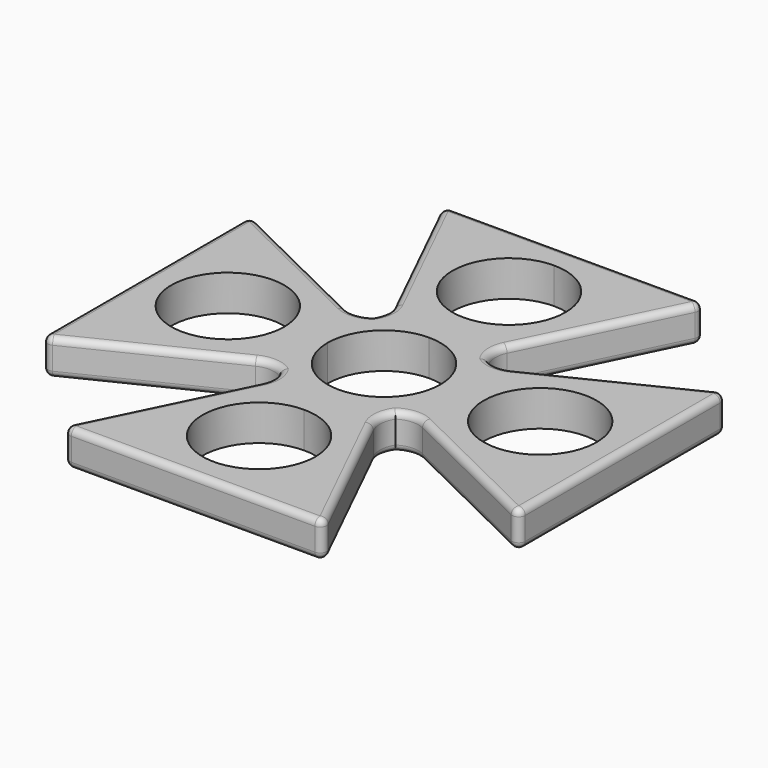
from build123d import *

# Parameters (mm, degrees)
F0_R          = 11.0109
F1_DEPTH      = 6.985
F2_R          = 1.27
F3_T1_DEPTH   = 6.985
F4_T1_DEPTH   = 47.5314771429
F4_T3_DEPTH   = 31.6719082331
F4_T5_DEPTH   = 31.6719082331
F4_T7_DEPTH   = 31.6719082331
F4_T9_DEPTH   = 47.5314771429
F4_T11_DEPTH  = 31.6719082331
F4_T13_DEPTH  = 31.6719082331
F4_T15_DEPTH  = 31.6719082331
F4_T17_DEPTH  = 31.6719082331
F4_T19_DEPTH  = 31.6719082331
F4_T22_ANGLE  = 116.1026378833
F4_T26_ANGLE  = 95.1309457851
F4_T31_ANGLE  = 95.1309457851
F4_S32_R      = 5.0800000002
F4_T33_DEPTH  = 7
F4_T35_ANGLE  = 116.1026378833
F4_T39_ANGLE  = 95.1309457851
F4_T44_ANGLE  = 95.1309457851
F4_S45_R      = 5.0800000002
F4_T46_DEPTH  = 8
F4_T48_ANGLE  = 116.1026378833
F4_T52_ANGLE  = 95.1309457851
F4_T57_ANGLE  = 95.1309457851
F4_S58_R      = 5.0800000002
F4_T59_DEPTH  = 8
F4_T61_ANGLE  = 116.1026378833
F4_T65_ANGLE  = 95.1309457851
F4_S66_R      = 5.0800000002
F4_T67_DEPTH  = 7
F4_T71_ANGLE  = 95.1309457851
F4_T76_ANGLE  = 95.1309457851
F4_S77_R      = 5.0800000002
F4_T78_DEPTH  = 8
F4_T82_ANGLE  = 95.1309457851
F4_T85_ANGLE  = 116.1026378833
F4_T87_ANGLE  = 116.1026378833
F4_T91_ANGLE  = 95.1309457851
F4_S92_R      = 5.0800000002
F4_T93_DEPTH  = 8
F4_T97_ANGLE  = 95.1309457851
F4_T100_ANGLE = 116.1026378833
F4_T102_ANGLE = 116.1026378833
F4_T106_ANGLE = 95.1309457851
F4_S107_R     = 5.0800000002
F4_T108_DEPTH = 8
F4_T112_ANGLE = 95.1309457851
F4_T117_ANGLE = 95.1309457851
F4_T122_ANGLE = 95.1309457851
F4_S123_R     = 5.0800000002
F4_T124_DEPTH = 8
F4_T129_ANGLE = 95.1309457851
F4_S131_R     = 5.0800000002
F4_T132_DEPTH = 7
F4_T135_ANGLE = 95.1309457851
F4_S137_R     = 5.0800000002
F4_T138_DEPTH = 7
F4_T144_ANGLE = 95.1309457851
F4_S145_R     = 5.0800000002
F4_T146_DEPTH = 8
F4_T150_ANGLE = 95.1309457851
F4_S152_R     = 5.0800000002
F4_T153_DEPTH = 8
F4_T159_ANGLE = 95.1309457851
F4_S161_R     = 5.0800000002
F4_T162_DEPTH = 8
F4_T165_ANGLE = 95.1309457851
F4_S167_R     = 5.0800000002
F4_T168_DEPTH = 8
F4_T174_ANGLE = 95.1309457851
F4_S176_R     = 5.0800000002
F4_T177_DEPTH = 8
F4_T180_ANGLE = 95.1309457851
F4_S182_R     = 5.0800000002
F4_T183_DEPTH = 8
F5_T1_DEPTH   = 31.6719082331
F5_T3_DEPTH   = 31.6719082331
F5_T5_DEPTH   = 31.6719082331
F5_T7_DEPTH   = 31.6719082331
F5_T9_DEPTH   = 47.5314771429
F5_T11_DEPTH  = 31.6719082331
F5_T13_DEPTH  = 31.6719082331
F5_T15_DEPTH  = 47.5314771429
F5_T17_DEPTH  = 31.6719082331
F5_T19_DEPTH  = 31.6719082331
F5_T22_ANGLE  = 116.1026378833
F5_T26_ANGLE  = 95.1309457851
F5_T31_ANGLE  = 95.1309457851
F5_S32_R      = 5.0800000002
F5_T33_DEPTH  = 8
F5_T35_ANGLE  = 116.1026378833
F5_T39_ANGLE  = 95.1309457851
F5_T44_ANGLE  = 95.1309457851
F5_S45_R      = 5.0800000002
F5_T46_DEPTH  = 8
F5_T48_ANGLE  = 116.1026378833
F5_T52_ANGLE  = 95.1309457851
F5_S53_R      = 5.0800000002
F5_T54_DEPTH  = 8
F5_T58_ANGLE  = 95.1309457851
F5_T63_ANGLE  = 95.1309457851
F5_T68_ANGLE  = 95.1309457851
F5_S69_R      = 5.0800000002
F5_T70_DEPTH  = 8
F5_T72_ANGLE  = 116.1026378833
F5_T74_ANGLE  = 116.1026378833
F5_T78_ANGLE  = 95.1309457851
F5_S79_R      = 5.0800000002
F5_T80_DEPTH  = 8
F5_T84_ANGLE  = 95.1309457851
F5_T89_ANGLE  = 95.1309457851
F5_T94_ANGLE  = 95.1309457851
F5_S95_R      = 5.0800000002
F5_T96_DEPTH  = 8
F5_T98_ANGLE  = 116.1026378833
F5_T102_ANGLE = 95.1309457851
F5_S103_R     = 5.0800000002
F5_T104_DEPTH = 8
F5_T108_ANGLE = 95.1309457851
F5_T111_ANGLE = 116.1026378833
F5_T115_ANGLE = 95.1309457851
F5_S116_R     = 5.0800000002
F5_T117_DEPTH = 8
F5_T121_ANGLE = 95.1309457851
F5_T124_ANGLE = 116.1026378833
F5_T129_ANGLE = 95.1309457851
F5_S131_R     = 5.0800000002
F5_T132_DEPTH = 8
F5_T135_ANGLE = 95.1309457851
F5_S136_R     = 5.0800000002
F5_T137_DEPTH = 8
F5_T144_ANGLE = 95.1309457851
F5_S146_R     = 5.0800000002
F5_T147_DEPTH = 8
F5_T150_ANGLE = 95.1309457851
F5_S151_R     = 5.0800000002
F5_T152_DEPTH = 8
F5_T159_ANGLE = 95.1309457851
F5_S160_R     = 5.0800000002
F5_T161_DEPTH = 8
F5_T165_ANGLE = 95.1309457851
F5_S166_R     = 5.0800000002
F5_T167_DEPTH = 8
F5_T174_ANGLE = 95.1309457851
F5_S176_R     = 5.0800000002
F5_T177_DEPTH = 8
F5_T180_ANGLE = 95.1309457851
F5_S181_R     = 5.0800000002
F5_T182_DEPTH = 8


# Not quite as in the source:
# - a fillet or chamfer that OpenCascade refuses, or shapes differently, is made with other operations: its cross-section is extruded or revolved along the edge and cut away or added


with BuildPart() as f1:
    # F0 (on Top) → F1 (new body)
    with BuildSketch(Plane.XY):
        with BuildLine():
            Line((15.875, 0), (11.0109, 0))
            ThreePointArc((11.0109, 0), (7.785882057, -7.785882057), (0, -11.0109))
            Line((0, -11.0109), (0, -15.875))
            ThreePointArc((0, -15.875), (4.8823009597, -15.1055871233), (9.2913414184, -12.8719306884))
            ThreePointArc((9.2913414184, -12.8719306884), (11.2253201513, -11.2253201513), (12.8719306884, -9.2913414184))
            ThreePointArc((12.8719306884, -9.2913414184), (15.1055871233, -4.8823009597), (15.875, 0))
        make_face()
        with BuildLine():
            ThreePointArc((0, 11.0109), (7.785882057, 7.785882057), (11.0109, 0))
            Line((11.0109, 0), (15.875, 0))
            ThreePointArc((15.875, 0), (15.1055871233, 4.8823009597), (12.8719306884, 9.2913414184))
            ThreePointArc((12.8719306884, 9.2913414184), (11.2253201513, 11.2253201513), (9.2913414184, 12.8719306884))
            ThreePointArc((9.2913414184, 12.8719306884), (4.8823009597, 15.1055871233), (0, 15.875))
            Line((0, 15.875), (0, 11.0109))
        make_face()
        with BuildLine():
            ThreePointArc((-11.0109, 0), (-7.785882057, 7.785882057), (0, 11.0109))
            Line((0, 11.0109), (0, 15.875))
            ThreePointArc((0, 15.875), (-4.8823009597, 15.1055871233), (-9.2913414184, 12.8719306884))
            ThreePointArc((-9.2913414184, 12.8719306884), (-11.2253201513, 11.2253201513), (-12.8719306884, 9.2913414184))
            ThreePointArc((-12.8719306884, 9.2913414184), (-15.1055871233, 4.8823009597), (-15.875, 0))
            Line((-15.875, 0), (-11.0109, 0))
        make_face()
        with BuildLine():
            Line((0, -15.875), (0, -11.0109))
            ThreePointArc((0, -11.0109), (-4.2136890054, -10.1727451445), (-7.785882057, -7.785882057))
            Line((-7.785882057, -7.785882057), (-11.2253201513, -11.2253201513))
            ThreePointArc((-11.2253201513, -11.2253201513), (-10.2913158565, -12.0873670807), (-9.2913414184, -12.8719306884))
            ThreePointArc((-9.2913414184, -12.8719306884), (-4.8823009597, -15.1055871233), (0, -15.875))
        make_face()
        with BuildLine():
            ThreePointArc((12.8719306884, 9.2913414184), (15.1055871233, 4.8823009597), (15.875, 0))
            ThreePointArc((15.875, 0), (15.1055871233, -4.8823009597), (12.8719306884, -9.2913414184))
            Line((12.8719306884, -9.2913414184), (46.5709, -25.8022200257))
            Line((46.5709, -25.8022200257), (46.5709, 25.8022200257))
            Line((46.5709, 25.8022200257), (12.8719306884, 9.2913414184))
        make_face()
        with BuildLine():
            ThreePointArc((41.4909, 0), (30.48, -11.0109), (19.4691, 0))
            ThreePointArc((19.4691, 0), (30.48, 11.0109), (41.4909, 0))
        make_face(mode=Mode.SUBTRACT)
        with BuildLine():
            ThreePointArc((-7.785882057, -7.785882057), (-10.1727451445, -4.2136890054), (-11.0109, 0))
            Line((-11.0109, 0), (-15.875, 0))
            ThreePointArc((-15.875, 0), (-15.1055871233, -4.8823009597), (-12.8719306884, -9.2913414184))
            ThreePointArc((-12.8719306884, -9.2913414184), (-12.0873670807, -10.2913158565), (-11.2253201513, -11.2253201513))
            Line((-11.2253201513, -11.2253201513), (-7.785882057, -7.785882057))
        make_face()
        with BuildLine():
            ThreePointArc((-9.2913414184, 12.8719306884), (-4.8823009597, 15.1055871233), (0, 15.875))
            Line((0, 15.875), (0, 19.4691))
            ThreePointArc((0, 19.4691), (-11.0109, 30.48), (0, 41.4909))
            Line((0, 41.4909), (0, 46.5709))
            Line((0, 46.5709), (-25.8022200257, 46.5709))
            Line((-25.8022200257, 46.5709), (-9.2913414184, 12.8719306884))
        make_face()
        with BuildLine():
            Line((0, 19.4691), (0, 15.875))
            ThreePointArc((0, 15.875), (4.8823009597, 15.1055871233), (9.2913414184, 12.8719306884))
            Line((9.2913414184, 12.8719306884), (25.8022200257, 46.5709))
            Line((25.8022200257, 46.5709), (0, 46.5709))
            Line((0, 46.5709), (0, 41.4909))
            ThreePointArc((0, 41.4909), (7.785882057, 38.265882057), (11.0109, 30.48))
            ThreePointArc((11.0109, 30.48), (7.785882057, 22.694117943), (0, 19.4691))
        make_face()
        with BuildLine():
            ThreePointArc((9.2913414184, -12.8719306884), (4.8823009597, -15.1055871233), (0, -15.875))
            ThreePointArc((0, -15.875), (-4.8823009597, -15.1055871233), (-9.2913414184, -12.8719306884))
            Line((-9.2913414184, -12.8719306884), (-25.8022200257, -46.5709))
            Line((-25.8022200257, -46.5709), (25.8022200257, -46.5709))
            Line((25.8022200257, -46.5709), (9.2913414184, -12.8719306884))
        make_face()
        with BuildLine():
            ThreePointArc((11.0109, -30.48), (-7.785882057, -38.265882057), (0, -19.4691))
            ThreePointArc((0, -19.4691), (7.785882057, -22.694117943), (11.0109, -30.48))
        make_face(mode=Mode.SUBTRACT)
        with BuildLine():
            ThreePointArc((-12.8719306884, -9.2913414184), (-15.1055871233, -4.8823009597), (-15.875, 0))
            ThreePointArc((-15.875, 0), (-15.1055871233, 4.8823009597), (-12.8719306884, 9.2913414184))
            Line((-12.8719306884, 9.2913414184), (-46.5709, 25.8022200257))
            Line((-46.5709, 25.8022200257), (-46.5709, -25.8022200257))
            Line((-46.5709, -25.8022200257), (-12.8719306884, -9.2913414184))
        make_face()
        with Locations((-30.48, 0)):
            Circle(F0_R, mode=Mode.SUBTRACT)
    extrude(amount=F1_DEPTH)

    # F2
    f2_edges = [f1.edges().sort_by_distance(p)[0] for p in [
        (-25.80222, 46.5709, 3.4925),
        (-46.5709, 25.80222, 3.4925),
        (25.80222, 46.5709, 3.4925),
        (46.5709, 25.80222, 3.4925),
        (-46.5709, -25.80222, 3.4925),
        (-25.80222, -46.5709, 3.4925),
        (25.80222, -46.5709, 3.4925),
        (46.5709, -25.80222, 3.4925),
    ]]
    fillet(f2_edges, radius=F2_R)

    # F3: fillet of radius 5.08 on 8 edges, made by hand

    # F3_s2 → F3_t1 (join)
    with BuildSketch(Plane.XY):
        with BuildLine():
            ThreePointArc((11.7674716509, 10.655619923), (10.5028634206, 13.3558434789), (10.971185393, 16.3005193113))
            Line((10.971185393, 16.3005193113), (9.2913414184, 12.8719306884))
            ThreePointArc((9.2913414184, 12.8719306884), (10.5875592241, 11.8287452705), (11.7674716509, 10.655619923))
        make_face()
        with BuildLine():
            ThreePointArc((16.3005193113, 10.971185393), (13.3558434789, 10.5028634206), (10.655619923, 11.7674716509))
            ThreePointArc((10.655619923, 11.7674716509), (11.8287452705, 10.5875592241), (12.8719306884, 9.2913414184))
            Line((12.8719306884, 9.2913414184), (16.3005193113, 10.971185393))
        make_face()
        with BuildLine():
            ThreePointArc((16.3005193113, -10.971185393), (13.3558434789, -10.5028634206), (10.655619923, -11.7674716509))
            ThreePointArc((10.655619923, -11.7674716509), (11.8287452705, -10.5875592241), (12.8719306884, -9.2913414184))
            Line((12.8719306884, -9.2913414184), (16.3005193113, -10.971185393))
        make_face()
        with BuildLine():
            ThreePointArc((11.7674716509, -10.655619923), (10.5028634206, -13.3558434789), (10.971185393, -16.3005193113))
            Line((10.971185393, -16.3005193113), (9.2913414184, -12.8719306884))
            ThreePointArc((9.2913414184, -12.8719306884), (10.5875592241, -11.8287452705), (11.7674716509, -10.655619923))
        make_face()
        with BuildLine():
            ThreePointArc((-10.971185393, -16.3005193113), (-10.5028634206, -13.3558434789), (-11.7674716509, -10.655619923))
            ThreePointArc((-11.7674716509, -10.655619923), (-10.5875592241, -11.8287452705), (-9.2913414184, -12.8719306884))
            Line((-9.2913414184, -12.8719306884), (-10.971185393, -16.3005193113))
        make_face()
        with BuildLine():
            ThreePointArc((-10.655619923, -11.7674716509), (-13.3558434789, -10.5028634206), (-16.3005193113, -10.971185393))
            Line((-16.3005193113, -10.971185393), (-12.8719306884, -9.2913414184))
            ThreePointArc((-12.8719306884, -9.2913414184), (-11.8287452705, -10.5875592241), (-10.655619923, -11.7674716509))
        make_face()
        with BuildLine():
            ThreePointArc((-10.655619923, 11.7674716509), (-13.3558434789, 10.5028634206), (-16.3005193113, 10.971185393))
            Line((-16.3005193113, 10.971185393), (-12.8719306884, 9.2913414184))
            ThreePointArc((-12.8719306884, 9.2913414184), (-11.8287452705, 10.5875592241), (-10.655619923, 11.7674716509))
        make_face()
        with BuildLine():
            ThreePointArc((-10.971185393, 16.3005193113), (-10.5028634206, 13.3558434789), (-11.7674716509, 10.655619923))
            ThreePointArc((-11.7674716509, 10.655619923), (-10.5875592241, 11.8287452705), (-9.2913414184, 12.8719306884))
            Line((-9.2913414184, 12.8719306884), (-10.971185393, 16.3005193113))
        make_face()
    extrude(amount=F3_T1_DEPTH)

    # F4: fillet of radius 1.27 on 4 edges, made by hand

    # F4_s2 → F4_t1 (cut)
    with BuildSketch(Plane.YZ.offset(-23.7657385714)):
        with BuildLine():
            ThreePointArc((-45.3009, 0), (-46.1989256121, 0.3719743879), (-46.5709, 1.27))
            Line((-46.5709, 1.27), (-46.5709, 0))
            Line((-46.5709, 0), (-45.3009, 0))
        make_face()
        with BuildLine():
            ThreePointArc((45.3009, 0), (46.1989256121, 0.3719743879), (46.5709, 1.27))
            Line((46.5709, 1.27), (46.5709, 0))
            Line((46.5709, 0), (45.3009, 0))
        make_face()
    extrude(amount=F4_T1_DEPTH, mode=Mode.SUBTRACT)

    # F4_s4 → F4_t3 (cut)
    with BuildSketch(Plane(origin=(-17.4797964099, 8.5642618305, 0), x_dir=(0, 0, 1), z_dir=(-0.8980073201, 0.4399805144, 0))):
        with BuildLine():
            ThreePointArc((0, 1.4102939225), (0.3719743879, 2.3083195346), (1.27, 2.6802939225))
            Line((1.27, 2.6802939225), (0, 2.6802939225))
            Line((0, 2.6802939225), (0, 1.4102939225))
        make_face()
    extrude(amount=F4_T3_DEPTH, mode=Mode.SUBTRACT)

    # F4_s6 → F4_t5 (cut)
    with BuildSketch(Plane(origin=(-22.4992843055, 45.9214018454, 0), x_dir=(0, 0, 1), z_dir=(0.4399805144, -0.8980073201, 0))):
        with BuildLine():
            ThreePointArc((0, 1.4102939225), (0.3719743879, 2.3083195346), (1.27, 2.6802939225))
            Line((1.27, 2.6802939225), (0, 2.6802939225))
            Line((0, 2.6802939225), (0, 1.4102939225))
        make_face()
    extrude(amount=F4_T5_DEPTH, mode=Mode.SUBTRACT)

    # F4_s8 → F4_t7 (cut)
    with BuildSketch(Plane(origin=(45.9214018454, 22.4992843055, 0), x_dir=(0, 0, 1), z_dir=(-0.8980073201, -0.4399805144, 0))):
        with BuildLine():
            ThreePointArc((0, 1.4102939225), (0.3719743879, 2.3083195346), (1.27, 2.6802939225))
            Line((1.27, 2.6802939225), (0, 2.6802939225))
            Line((0, 2.6802939225), (0, 1.4102939225))
        make_face()
    extrude(amount=F4_T7_DEPTH, mode=Mode.SUBTRACT)

    # F4_s10 → F4_t9 (cut)
    with BuildSketch(Plane.XZ.offset(-23.7657385714)):
        with BuildLine():
            ThreePointArc((45.3009, 0), (46.1989256121, 0.3719743879), (46.5709, 1.27))
            Line((46.5709, 1.27), (46.5709, 0))
            Line((46.5709, 0), (45.3009, 0))
        make_face()
        with BuildLine():
            ThreePointArc((-45.3009, 0), (-46.1989256121, 0.3719743879), (-46.5709, 1.27))
            Line((-46.5709, 1.27), (-46.5709, 0))
            Line((-46.5709, 0), (-45.3009, 0))
        make_face()
    extrude(amount=F4_T9_DEPTH, mode=Mode.SUBTRACT)

    # F4_s12 → F4_t11 (cut)
    with BuildSketch(Plane(origin=(17.4797964099, -8.5642618305, 0), x_dir=(0, 0, 1), z_dir=(0.8980073201, -0.4399805144, 0))):
        with BuildLine():
            ThreePointArc((1.27, 2.6802939225), (0.3719743879, 2.3083195346), (0, 1.4102939225))
            Line((0, 1.4102939225), (0, 2.6802939225))
            Line((0, 2.6802939225), (1.27, 2.6802939225))
        make_face()
    extrude(amount=F4_T11_DEPTH, mode=Mode.SUBTRACT)

    # F4_s14 → F4_t13 (cut)
    with BuildSketch(Plane(origin=(8.5642618305, 17.4797964099, 0), x_dir=(0, 0, 1), z_dir=(0.4399805144, 0.8980073201, 0))):
        with BuildLine():
            ThreePointArc((0, 1.4102939225), (0.3719743879, 2.3083195346), (1.27, 2.6802939225))
            Line((1.27, 2.6802939225), (0, 2.6802939225))
            Line((0, 2.6802939225), (0, 1.4102939225))
        make_face()
    extrude(amount=F4_T13_DEPTH, mode=Mode.SUBTRACT)

    # F4_s16 → F4_t15 (cut)
    with BuildSketch(Plane(origin=(-45.9214018454, -22.4992843055, 0), x_dir=(0, 0, 1), z_dir=(0.8980073201, 0.4399805144, 0))):
        with BuildLine():
            ThreePointArc((0, 1.4102939225), (0.3719743879, 2.3083195346), (1.27, 2.6802939225))
            Line((1.27, 2.6802939225), (0, 2.6802939225))
            Line((0, 2.6802939225), (0, 1.4102939225))
        make_face()
    extrude(amount=F4_T15_DEPTH, mode=Mode.SUBTRACT)

    # F4_s18 → F4_t17 (cut)
    with BuildSketch(Plane(origin=(22.4992843055, -45.9214018454, 0), x_dir=(0, 0, 1), z_dir=(-0.4399805144, 0.8980073201, 0))):
        with BuildLine():
            ThreePointArc((0, 1.4102939225), (0.3719743879, 2.3083195346), (1.27, 2.6802939225))
            Line((1.27, 2.6802939225), (0, 2.6802939225))
            Line((0, 2.6802939225), (0, 1.4102939225))
        make_face()
    extrude(amount=F4_T17_DEPTH, mode=Mode.SUBTRACT)

    # F4_s20 → F4_t19 (cut)
    with BuildSketch(Plane(origin=(-8.5642618305, -17.4797964099, 0), x_dir=(0, 0, 1), z_dir=(-0.4399805144, -0.8980073201, 0))):
        with BuildLine():
            ThreePointArc((0, 1.4102939225), (0.3719743879, 2.3083195346), (1.27, 2.6802939225))
            Line((1.27, 2.6802939225), (0, 2.6802939225))
            Line((0, 2.6802939225), (0, 1.4102939225))
        make_face()
    extrude(amount=F4_T19_DEPTH, mode=Mode.SUBTRACT)

    # F4_s21 → F4_t22 (revolve, cut)
    with BuildSketch(Plane.XZ.offset(-23.7657385714)):
        with BuildLine():
            ThreePointArc((45.3009, 0), (46.1989256121, 0.3719743879), (46.5709, 1.27))
            Line((46.5709, 1.27), (46.5709, 0))
            Line((46.5709, 0), (45.3009, 0))
        make_face()
    revolve(axis=Axis((45.3009, 23.7657385714, 0), (0, 0, 1)), revolution_arc=F4_T22_ANGLE, mode=Mode.SUBTRACT)


with BuildPart() as f4_tool24:
    # F4_s25 → F4_t26 (revolve)
    with BuildSketch(Plane(origin=(17.4797964101, 8.5642618302, 0), x_dir=(0, 0, 1), z_dir=(0.8980073201, 0.4399805143, 0))):
        with BuildLine():
            ThreePointArc((0, -1.4102939229), (0.3719743879, -2.308319535), (1.27, -2.6802939229))
            Line((1.27, -2.6802939229), (0, -2.6802939229))
            Line((0, -2.6802939229), (0, -1.4102939229))
        make_face()
    revolve(axis=Axis((14.0654182984, 15.5330625794, 0), (0, 0, -1)), revolution_arc=F4_T26_ANGLE)

    split(bisect_by=Plane(origin=(-1.1792770986, 2.4069235625, 0), x_dir=(0, 0, 1), z_dir=(0.4399805144, -0.8980073201, 0)), keep=Keep.TOP)


with BuildPart() as f1_1:
    add(f1.part)

    # F4_t23: cut F4_tool24
    add(f4_tool24.part, mode=Mode.SUBTRACT)


with BuildPart() as f4_tool29:
    # F4_s30 → F4_t31 (revolve)
    with BuildSketch(Plane(origin=(17.4797964101, 8.5642618302, 0), x_dir=(0, 0, 1), z_dir=(0.8980073201, 0.4399805143, 0))):
        with BuildLine():
            ThreePointArc((0, -1.4102939229), (0.3719743879, -2.308319535), (1.27, -2.6802939229))
            Line((1.27, -2.6802939229), (0, -2.6802939229))
            Line((0, -2.6802939229), (0, -1.4102939229))
        make_face()
    revolve(axis=Axis((14.0654182984, 15.5330625794, 0), (0, 0, -1)), revolution_arc=F4_T31_ANGLE)

    # F4_s32 → F4_t33 (intersect, symmetric)
    with BuildSketch(Plane.XY.offset(1.1)):
        with Locations((15.5330625794, 14.0654182984)):
            Circle(F4_S32_R)
    extrude(amount=F4_T33_DEPTH, both=True, mode=Mode.INTERSECT)


with BuildPart() as f1_2:
    add(f1_1.part)

    # F4_t28: cut F4_tool29
    add(f4_tool29.part, mode=Mode.SUBTRACT)

    # F4_s34 → F4_t35 (revolve, cut)
    with BuildSketch(Plane(origin=(45.9214018454, -22.4992843055, 0), x_dir=(0, 0, 1), z_dir=(-0.8980073201, 0.4399805144, 0))):
        with BuildLine():
            ThreePointArc((0, -1.4102939225), (0.3719743879, -2.3083195346), (1.27, -2.6802939225))
            Line((1.27, -2.6802939225), (0, -2.6802939225))
            Line((0, -2.6802939225), (0, -1.4102939225))
        make_face()
    revolve(axis=Axis((45.3009, -23.7657385714, 0), (0, 0, 1)), revolution_arc=F4_T35_ANGLE, mode=Mode.SUBTRACT)


with BuildPart() as f4_tool37:
    # F4_s38 → F4_t39 (revolve)
    with BuildSketch(Plane(origin=(17.4797964101, -8.5642618302, 0), x_dir=(0, 0, 1), z_dir=(0.8980073201, -0.4399805143, 0))):
        with BuildLine():
            ThreePointArc((0, 1.4102939229), (0.3719743879, 2.308319535), (1.27, 2.6802939229))
            Line((1.27, 2.6802939229), (0, 2.6802939229))
            Line((0, 2.6802939229), (0, 1.4102939229))
        make_face()
    revolve(axis=Axis((14.0654182984, -15.5330625794, 0), (0, 0, 1)), revolution_arc=F4_T39_ANGLE)

    split(bisect_by=Plane(origin=(-1.1792770986, -2.4069235625, 0), x_dir=(0, 0, 1), z_dir=(0.4399805144, 0.8980073201, 0)), keep=Keep.TOP)


with BuildPart() as f1_3:
    add(f1_2.part)

    # F4_t36: cut F4_tool37
    add(f4_tool37.part, mode=Mode.SUBTRACT)


with BuildPart() as f4_tool42:
    # F4_s43 → F4_t44 (revolve)
    with BuildSketch(Plane(origin=(17.4797964101, -8.5642618302, 0), x_dir=(0, 0, 1), z_dir=(0.8980073201, -0.4399805143, 0))):
        with BuildLine():
            ThreePointArc((0, 1.4102939229), (0.3719743879, 2.308319535), (1.27, 2.6802939229))
            Line((1.27, 2.6802939229), (0, 2.6802939229))
            Line((0, 2.6802939229), (0, 1.4102939229))
        make_face()
    revolve(axis=Axis((14.0654182984, -15.5330625794, 0), (0, 0, 1)), revolution_arc=F4_T44_ANGLE)

    # F4_s45 → F4_t46 (intersect, symmetric)
    with BuildSketch(Plane.XY.offset(1.1)):
        with Locations((15.5330625794, -14.0654182984)):
            Circle(F4_S45_R)
    extrude(amount=F4_T46_DEPTH, both=True, mode=Mode.INTERSECT)


with BuildPart() as f1_4:
    add(f1_3.part)

    # F4_t41: cut F4_tool42
    add(f4_tool42.part, mode=Mode.SUBTRACT)

    # F4_s47 → F4_t48 (revolve, cut)
    with BuildSketch(Plane.YZ.offset(-23.7657385714)):
        with BuildLine():
            ThreePointArc((45.3009, 0), (46.1989256121, 0.3719743879), (46.5709, 1.27))
            Line((46.5709, 1.27), (46.5709, 0))
            Line((46.5709, 0), (45.3009, 0))
        make_face()
    revolve(axis=Axis((-23.7657385714, 45.3009, 0), (0, 0, 1)), revolution_arc=F4_T48_ANGLE, mode=Mode.SUBTRACT)


with BuildPart() as f4_tool50:
    # F4_s51 → F4_t52 (revolve)
    with BuildSketch(Plane(origin=(-8.5642618302, 17.4797964101, 0), x_dir=(0, 0, 1), z_dir=(-0.4399805143, 0.8980073201, 0))):
        with BuildLine():
            ThreePointArc((0, -1.4102939229), (0.3719743879, -2.308319535), (1.27, -2.6802939229))
            Line((1.27, -2.6802939229), (0, -2.6802939229))
            Line((0, -2.6802939229), (0, -1.4102939229))
        make_face()
    revolve(axis=Axis((-15.5330625794, 14.0654182984, 0), (0, 0, -1)), revolution_arc=F4_T52_ANGLE)

    split(bisect_by=Plane(origin=(-2.4069235625, -1.1792770986, 0), x_dir=(0, 0, 1), z_dir=(0.8980073201, 0.4399805144, 0)), keep=Keep.TOP)


with BuildPart() as f1_5:
    add(f1_4.part)

    # F4_t49: cut F4_tool50
    add(f4_tool50.part, mode=Mode.SUBTRACT)


with BuildPart() as f4_tool55:
    # F4_s56 → F4_t57 (revolve)
    with BuildSketch(Plane(origin=(-8.5642618302, 17.4797964101, 0), x_dir=(0, 0, 1), z_dir=(-0.4399805143, 0.8980073201, 0))):
        with BuildLine():
            ThreePointArc((0, -1.4102939229), (0.3719743879, -2.308319535), (1.27, -2.6802939229))
            Line((1.27, -2.6802939229), (0, -2.6802939229))
            Line((0, -2.6802939229), (0, -1.4102939229))
        make_face()
    revolve(axis=Axis((-15.5330625794, 14.0654182984, 0), (0, 0, -1)), revolution_arc=F4_T57_ANGLE)

    # F4_s58 → F4_t59 (intersect, symmetric)
    with BuildSketch(Plane.XY.offset(1.1)):
        with Locations((-14.0654182984, 15.5330625794)):
            Circle(F4_S58_R)
    extrude(amount=F4_T59_DEPTH, both=True, mode=Mode.INTERSECT)


with BuildPart() as f1_6:
    add(f1_5.part)

    # F4_t54: cut F4_tool55
    add(f4_tool55.part, mode=Mode.SUBTRACT)

    # F4_s60 → F4_t61 (revolve, cut)
    with BuildSketch(Plane(origin=(22.4992843055, 45.9214018454, 0), x_dir=(0, 0, 1), z_dir=(-0.4399805144, -0.8980073201, 0))):
        with BuildLine():
            ThreePointArc((0, -1.4102939225), (0.3719743879, -2.3083195346), (1.27, -2.6802939225))
            Line((1.27, -2.6802939225), (0, -2.6802939225))
            Line((0, -2.6802939225), (0, -1.4102939225))
        make_face()
    revolve(axis=Axis((23.7657385714, 45.3009, 0), (0, 0, 1)), revolution_arc=F4_T61_ANGLE, mode=Mode.SUBTRACT)


with BuildPart() as f4_tool63:
    # F4_s64 → F4_t65 (revolve)
    with BuildSketch(Plane(origin=(8.8426868158, -3.3893777596, 0), x_dir=(0, 0, 1), z_dir=(0.93375737, -0.3579066554, 0))):
        with BuildLine():
            ThreePointArc((0, -12.3430744737), (0.3719743879, -13.2411000858), (1.27, -13.6130744737))
            Line((1.27, -13.6130744737), (0, -13.6130744737))
            Line((0, -13.6130744737), (0, -12.3430744737))
        make_face()
    revolve(axis=Axis((15.5330625794, 14.0654182984, 0), (0, 0, -1)), revolution_arc=F4_T65_ANGLE)

    # F4_s66 → F4_t67 (intersect, symmetric)
    with BuildSketch(Plane.XY.offset(1.1)):
        with Locations((14.0654182984, 15.5330625794)):
            Circle(F4_S66_R)
    extrude(amount=F4_T67_DEPTH, both=True, mode=Mode.INTERSECT)


with BuildPart() as f1_7:
    add(f1_6.part)

    # F4_t62: cut F4_tool63
    add(f4_tool63.part, mode=Mode.SUBTRACT)


with BuildPart() as f4_tool69:
    # F4_s70 → F4_t71 (revolve)
    with BuildSketch(Plane(origin=(8.8426868158, -3.3893777596, 0), x_dir=(0, 0, 1), z_dir=(0.93375737, -0.3579066554, 0))):
        with BuildLine():
            ThreePointArc((0, -12.3430744737), (0.3719743879, -13.2411000858), (1.27, -13.6130744737))
            Line((1.27, -13.6130744737), (0, -13.6130744737))
            Line((0, -13.6130744737), (0, -12.3430744737))
        make_face()
    revolve(axis=Axis((15.5330625794, 14.0654182984, 0), (0, 0, -1)), revolution_arc=F4_T71_ANGLE)

    split(bisect_by=Plane(origin=(2.4069235625, -1.1792770986, 0), x_dir=(0, 0, 1), z_dir=(-0.8980073201, 0.4399805144, 0)), keep=Keep.TOP)


with BuildPart() as f1_8:
    add(f1_7.part)

    # F4_t68: cut F4_tool69
    add(f4_tool69.part, mode=Mode.SUBTRACT)


with BuildPart() as f4_tool74:
    # F4_s75 → F4_t76 (revolve)
    with BuildSketch(Plane(origin=(3.3893777596, 8.8426868158, 0), x_dir=(0, 0, 1), z_dir=(0.3579066554, 0.93375737, 0))):
        with BuildLine():
            ThreePointArc((0, -12.3430744737), (0.3719743879, -13.2411000858), (1.27, -13.6130744737))
            Line((1.27, -13.6130744737), (0, -13.6130744737))
            Line((0, -13.6130744737), (0, -12.3430744737))
        make_face()
    revolve(axis=Axis((-14.0654182984, 15.5330625794, 0), (0, 0, -1)), revolution_arc=F4_T76_ANGLE)

    # F4_s77 → F4_t78 (intersect, symmetric)
    with BuildSketch(Plane.XY.offset(1.1)):
        with Locations((-15.5330625794, 14.0654182984)):
            Circle(F4_S77_R)
    extrude(amount=F4_T78_DEPTH, both=True, mode=Mode.INTERSECT)


with BuildPart() as f1_9:
    add(f1_8.part)

    # F4_t73: cut F4_tool74
    add(f4_tool74.part, mode=Mode.SUBTRACT)


with BuildPart() as f4_tool80:
    # F4_s81 → F4_t82 (revolve)
    with BuildSketch(Plane(origin=(3.3893777596, 8.8426868158, 0), x_dir=(0, 0, 1), z_dir=(0.3579066554, 0.93375737, 0))):
        with BuildLine():
            ThreePointArc((0, -12.3430744737), (0.3719743879, -13.2411000858), (1.27, -13.6130744737))
            Line((1.27, -13.6130744737), (0, -13.6130744737))
            Line((0, -13.6130744737), (0, -12.3430744737))
        make_face()
    revolve(axis=Axis((-14.0654182984, 15.5330625794, 0), (0, 0, -1)), revolution_arc=F4_T82_ANGLE)

    split(bisect_by=Plane(origin=(1.1792770986, 2.4069235625, 0), x_dir=(0, 0, 1), z_dir=(-0.4399805144, -0.8980073201, 0)), keep=Keep.TOP)


with BuildPart() as f1_10:
    add(f1_9.part)

    # F4_t79: cut F4_tool80
    add(f4_tool80.part, mode=Mode.SUBTRACT)

    # F4_s84 → F4_t85 (revolve, cut)
    with BuildSketch(Plane(origin=(-45.9214018454, 22.4992843055, 0), x_dir=(0, 0, 1), z_dir=(0.8980073201, -0.4399805144, 0))):
        with BuildLine():
            ThreePointArc((0, -1.4102939225), (0.3719743879, -2.3083195346), (1.27, -2.6802939225))
            Line((1.27, -2.6802939225), (0, -2.6802939225))
            Line((0, -2.6802939225), (0, -1.4102939225))
        make_face()
    revolve(axis=Axis((-45.3009, 23.7657385714, 0), (0, 0, 1)), revolution_arc=F4_T85_ANGLE, mode=Mode.SUBTRACT)

    # F4_s86 → F4_t87 (revolve, cut)
    with BuildSketch(Plane.XZ.offset(23.7657385714)):
        with BuildLine():
            ThreePointArc((-45.3009, 0), (-46.1989256121, 0.3719743879), (-46.5709, 1.27))
            Line((-46.5709, 1.27), (-46.5709, 0))
            Line((-46.5709, 0), (-45.3009, 0))
        make_face()
    revolve(axis=Axis((-45.3009, -23.7657385714, 0), (0, 0, 1)), revolution_arc=F4_T87_ANGLE, mode=Mode.SUBTRACT)


with BuildPart() as f4_tool89:
    # F4_s90 → F4_t91 (revolve)
    with BuildSketch(Plane(origin=(3.3893777596, -8.8426868158, 0), x_dir=(0, 0, 1), z_dir=(0.3579066554, -0.93375737, 0))):
        with BuildLine():
            ThreePointArc((0, 12.3430744737), (0.3719743879, 13.2411000858), (1.27, 13.6130744737))
            Line((1.27, 13.6130744737), (0, 13.6130744737))
            Line((0, 13.6130744737), (0, 12.3430744737))
        make_face()
    revolve(axis=Axis((-14.0654182984, -15.5330625794, 0), (0, 0, 1)), revolution_arc=F4_T91_ANGLE)

    # F4_s92 → F4_t93 (intersect, symmetric)
    with BuildSketch(Plane.XY.offset(1.1)):
        with Locations((-15.5330625794, -14.0654182984)):
            Circle(F4_S92_R)
    extrude(amount=F4_T93_DEPTH, both=True, mode=Mode.INTERSECT)


with BuildPart() as f1_11:
    add(f1_10.part)

    # F4_t88: cut F4_tool89
    add(f4_tool89.part, mode=Mode.SUBTRACT)


with BuildPart() as f4_tool95:
    # F4_s96 → F4_t97 (revolve)
    with BuildSketch(Plane(origin=(3.3893777596, -8.8426868158, 0), x_dir=(0, 0, 1), z_dir=(0.3579066554, -0.93375737, 0))):
        with BuildLine():
            ThreePointArc((0, 12.3430744737), (0.3719743879, 13.2411000858), (1.27, 13.6130744737))
            Line((1.27, 13.6130744737), (0, 13.6130744737))
            Line((0, 13.6130744737), (0, 12.3430744737))
        make_face()
    revolve(axis=Axis((-14.0654182984, -15.5330625794, 0), (0, 0, 1)), revolution_arc=F4_T97_ANGLE)

    split(bisect_by=Plane(origin=(1.1792770986, -2.4069235625, 0), x_dir=(0, 0, 1), z_dir=(-0.4399805144, 0.8980073201, 0)), keep=Keep.TOP)


with BuildPart() as f1_12:
    add(f1_11.part)

    # F4_t94: cut F4_tool95
    add(f4_tool95.part, mode=Mode.SUBTRACT)

    # F4_s99 → F4_t100 (revolve, cut)
    with BuildSketch(Plane(origin=(-22.4992843055, -45.9214018454, 0), x_dir=(0, 0, 1), z_dir=(0.4399805144, 0.8980073201, 0))):
        with BuildLine():
            ThreePointArc((0, -1.4102939225), (0.3719743879, -2.3083195346), (1.27, -2.6802939225))
            Line((1.27, -2.6802939225), (0, -2.6802939225))
            Line((0, -2.6802939225), (0, -1.4102939225))
        make_face()
    revolve(axis=Axis((-23.7657385714, -45.3009, 0), (0, 0, 1)), revolution_arc=F4_T100_ANGLE, mode=Mode.SUBTRACT)

    # F4_s101 → F4_t102 (revolve, cut)
    with BuildSketch(Plane.YZ.offset(23.7657385714)):
        with BuildLine():
            ThreePointArc((-45.3009, 0), (-46.1989256121, 0.3719743879), (-46.5709, 1.27))
            Line((-46.5709, 1.27), (-46.5709, 0))
            Line((-46.5709, 0), (-45.3009, 0))
        make_face()
    revolve(axis=Axis((23.7657385714, -45.3009, 0), (0, 0, 1)), revolution_arc=F4_T102_ANGLE, mode=Mode.SUBTRACT)


with BuildPart() as f4_tool104:
    # F4_s105 → F4_t106 (revolve)
    with BuildSketch(Plane(origin=(8.8426868158, 3.3893777596, 0), x_dir=(0, 0, 1), z_dir=(0.93375737, 0.3579066554, 0))):
        with BuildLine():
            ThreePointArc((0, 12.3430744737), (0.3719743879, 13.2411000858), (1.27, 13.6130744737))
            Line((1.27, 13.6130744737), (0, 13.6130744737))
            Line((0, 13.6130744737), (0, 12.3430744737))
        make_face()
    revolve(axis=Axis((15.5330625794, -14.0654182984, 0), (0, 0, 1)), revolution_arc=F4_T106_ANGLE)

    # F4_s107 → F4_t108 (intersect, symmetric)
    with BuildSketch(Plane.XY.offset(1.1)):
        with Locations((14.0654182984, -15.5330625794)):
            Circle(F4_S107_R)
    extrude(amount=F4_T108_DEPTH, both=True, mode=Mode.INTERSECT)


with BuildPart() as f1_13:
    add(f1_12.part)

    # F4_t103: cut F4_tool104
    add(f4_tool104.part, mode=Mode.SUBTRACT)


with BuildPart() as f4_tool110:
    # F4_s111 → F4_t112 (revolve)
    with BuildSketch(Plane(origin=(8.8426868158, 3.3893777596, 0), x_dir=(0, 0, 1), z_dir=(0.93375737, 0.3579066554, 0))):
        with BuildLine():
            ThreePointArc((0, 12.3430744737), (0.3719743879, 13.2411000858), (1.27, 13.6130744737))
            Line((1.27, 13.6130744737), (0, 13.6130744737))
            Line((0, 13.6130744737), (0, 12.3430744737))
        make_face()
    revolve(axis=Axis((15.5330625794, -14.0654182984, 0), (0, 0, 1)), revolution_arc=F4_T112_ANGLE)

    split(bisect_by=Plane(origin=(2.4069235625, 1.1792770986, 0), x_dir=(0, 0, 1), z_dir=(-0.8980073201, -0.4399805144, 0)), keep=Keep.TOP)


with BuildPart() as f1_14:
    add(f1_13.part)

    # F4_t109: cut F4_tool110
    add(f4_tool110.part, mode=Mode.SUBTRACT)


with BuildPart() as f4_tool115:
    # F4_s116 → F4_t117 (revolve)
    with BuildSketch(Plane(origin=(-8.5642618302, -17.4797964101, 0), x_dir=(0, 0, 1), z_dir=(-0.4399805143, -0.8980073201, 0))):
        with BuildLine():
            ThreePointArc((0, 1.4102939229), (0.3719743879, 2.308319535), (1.27, 2.6802939229))
            Line((1.27, 2.6802939229), (0, 2.6802939229))
            Line((0, 2.6802939229), (0, 1.4102939229))
        make_face()
    revolve(axis=Axis((-15.5330625794, -14.0654182984, 0), (0, 0, 1)), revolution_arc=F4_T117_ANGLE)

    split(bisect_by=Plane(origin=(-2.4069235625, 1.1792770986, 0), x_dir=(0, 0, 1), z_dir=(0.8980073201, -0.4399805144, 0)), keep=Keep.TOP)


with BuildPart() as f1_15:
    add(f1_14.part)

    # F4_t114: cut F4_tool115
    add(f4_tool115.part, mode=Mode.SUBTRACT)


with BuildPart() as f4_tool120:
    # F4_s121 → F4_t122 (revolve)
    with BuildSketch(Plane(origin=(-8.5642618302, -17.4797964101, 0), x_dir=(0, 0, 1), z_dir=(-0.4399805143, -0.8980073201, 0))):
        with BuildLine():
            ThreePointArc((0, 1.4102939229), (0.3719743879, 2.308319535), (1.27, 2.6802939229))
            Line((1.27, 2.6802939229), (0, 2.6802939229))
            Line((0, 2.6802939229), (0, 1.4102939229))
        make_face()
    revolve(axis=Axis((-15.5330625794, -14.0654182984, 0), (0, 0, 1)), revolution_arc=F4_T122_ANGLE)

    # F4_s123 → F4_t124 (intersect, symmetric)
    with BuildSketch(Plane.XY.offset(1.1)):
        with Locations((-14.0654182984, -15.5330625794)):
            Circle(F4_S123_R)
    extrude(amount=F4_T124_DEPTH, both=True, mode=Mode.INTERSECT)


with BuildPart() as f1_16:
    add(f1_15.part)

    # F4_t119: cut F4_tool120
    add(f4_tool120.part, mode=Mode.SUBTRACT)


with BuildPart() as f4_tool127:
    # F4_s128 → F4_t129 (revolve)
    with BuildSketch(Plane(origin=(17.4797964101, 8.5642618302, 0), x_dir=(0, 0, 1), z_dir=(0.8980073201, 0.4399805143, 0))):
        with BuildLine():
            ThreePointArc((0, -1.4102939229), (0.3719743879, -2.308319535), (1.27, -2.6802939229))
            Line((1.27, -2.6802939229), (0, -2.6802939229))
            Line((0, -2.6802939229), (0, -1.4102939229))
        make_face()
    revolve(axis=Axis((14.0654182984, 15.5330625794, 0), (0, 0, -1)), revolution_arc=F4_T129_ANGLE)

    split(bisect_by=Plane(origin=(-1.1792770986, 2.4069235625, 0), x_dir=(0, 0, 1), z_dir=(-0.4399805144, 0.8980073201, 0)), keep=Keep.TOP)

    # F4_s131 → F4_t132 (cut, symmetric)
    with BuildSketch(Plane.XY.offset(1.1)):
        with Locations((15.5330625794, 14.0654182984)):
            Circle(F4_S131_R)
    extrude(amount=F4_T132_DEPTH, both=True, mode=Mode.SUBTRACT)


with BuildPart() as f4_tool133:
    # F4_s134 → F4_t135 (revolve)
    with BuildSketch(Plane(origin=(8.8426868158, -3.3893777596, 0), x_dir=(0, 0, 1), z_dir=(0.93375737, -0.3579066554, 0))):
        with BuildLine():
            ThreePointArc((0, -12.3430744737), (0.3719743879, -13.2411000858), (1.27, -13.6130744737))
            Line((1.27, -13.6130744737), (0, -13.6130744737))
            Line((0, -13.6130744737), (0, -12.3430744737))
        make_face()
    revolve(axis=Axis((15.5330625794, 14.0654182984, 0), (0, 0, -1)), revolution_arc=F4_T135_ANGLE)

    split(bisect_by=Plane(origin=(2.4069235625, -1.1792770986, 0), x_dir=(0, 0, 1), z_dir=(0.8980073201, -0.4399805144, 0)), keep=Keep.TOP)

    # F4_s137 → F4_t138 (cut, symmetric)
    with BuildSketch(Plane.XY.offset(1.1)):
        with Locations((14.0654182984, 15.5330625794)):
            Circle(F4_S137_R)
    extrude(amount=F4_T138_DEPTH, both=True, mode=Mode.SUBTRACT)


with BuildPart() as f4_tool127_1:
    add(f4_tool127.part)

    # F4_t139: intersect F4_tool133
    add(f4_tool133.part, mode=Mode.INTERSECT)


with BuildPart() as f1_17:
    add(f1_16.part)

    # F4_t125: cut F4_tool127
    add(f4_tool127_1.part, mode=Mode.SUBTRACT)


with BuildPart() as f4_tool142:
    # F4_s143 → F4_t144 (revolve)
    with BuildSketch(Plane(origin=(8.8426868158, 3.3893777596, 0), x_dir=(0, 0, 1), z_dir=(0.93375737, 0.3579066554, 0))):
        with BuildLine():
            ThreePointArc((0, 12.3430744737), (0.3719743879, 13.2411000858), (1.27, 13.6130744737))
            Line((1.27, 13.6130744737), (0, 13.6130744737))
            Line((0, 13.6130744737), (0, 12.3430744737))
        make_face()
    revolve(axis=Axis((15.5330625794, -14.0654182984, 0), (0, 0, 1)), revolution_arc=F4_T144_ANGLE)

    # F4_s145 → F4_t146 (cut, symmetric)
    with BuildSketch(Plane.XY.offset(1.1)):
        with Locations((14.0654182984, -15.5330625794)):
            Circle(F4_S145_R)
    extrude(amount=F4_T146_DEPTH, both=True, mode=Mode.SUBTRACT)

    split(bisect_by=Plane(origin=(2.4069235625, 1.1792770986, 0), x_dir=(0, 0, 1), z_dir=(0.8980073201, 0.4399805144, 0)), keep=Keep.TOP)


with BuildPart() as f4_tool148:
    # F4_s149 → F4_t150 (revolve)
    with BuildSketch(Plane(origin=(17.4797964101, -8.5642618302, 0), x_dir=(0, 0, 1), z_dir=(0.8980073201, -0.4399805143, 0))):
        with BuildLine():
            ThreePointArc((0, 1.4102939229), (0.3719743879, 2.308319535), (1.27, 2.6802939229))
            Line((1.27, 2.6802939229), (0, 2.6802939229))
            Line((0, 2.6802939229), (0, 1.4102939229))
        make_face()
    revolve(axis=Axis((14.0654182984, -15.5330625794, 0), (0, 0, 1)), revolution_arc=F4_T150_ANGLE)

    split(bisect_by=Plane(origin=(-1.1792770986, -2.4069235625, 0), x_dir=(0, 0, 1), z_dir=(-0.4399805144, -0.8980073201, 0)), keep=Keep.TOP)

    # F4_s152 → F4_t153 (cut, symmetric)
    with BuildSketch(Plane.XY.offset(1.1)):
        with Locations((15.5330625794, -14.0654182984)):
            Circle(F4_S152_R)
    extrude(amount=F4_T153_DEPTH, both=True, mode=Mode.SUBTRACT)


with BuildPart() as f4_tool142_1:
    add(f4_tool142.part)

    # F4_t154: intersect F4_tool148
    add(f4_tool148.part, mode=Mode.INTERSECT)


with BuildPart() as f1_18:
    add(f1_17.part)

    # F4_t140: cut F4_tool142
    add(f4_tool142_1.part, mode=Mode.SUBTRACT)


with BuildPart() as f4_tool157:
    # F4_s158 → F4_t159 (revolve)
    with BuildSketch(Plane(origin=(-8.5642618302, 17.4797964101, 0), x_dir=(0, 0, 1), z_dir=(-0.4399805143, 0.8980073201, 0))):
        with BuildLine():
            ThreePointArc((0, -1.4102939229), (0.3719743879, -2.308319535), (1.27, -2.6802939229))
            Line((1.27, -2.6802939229), (0, -2.6802939229))
            Line((0, -2.6802939229), (0, -1.4102939229))
        make_face()
    revolve(axis=Axis((-15.5330625794, 14.0654182984, 0), (0, 0, -1)), revolution_arc=F4_T159_ANGLE)

    split(bisect_by=Plane(origin=(-2.4069235625, -1.1792770986, 0), x_dir=(0, 0, 1), z_dir=(-0.8980073201, -0.4399805144, 0)), keep=Keep.TOP)

    # F4_s161 → F4_t162 (cut, symmetric)
    with BuildSketch(Plane.XY.offset(1.1)):
        with Locations((-14.0654182984, 15.5330625794)):
            Circle(F4_S161_R)
    extrude(amount=F4_T162_DEPTH, both=True, mode=Mode.SUBTRACT)


with BuildPart() as f4_tool163:
    # F4_s164 → F4_t165 (revolve)
    with BuildSketch(Plane(origin=(3.3893777596, 8.8426868158, 0), x_dir=(0, 0, 1), z_dir=(0.3579066554, 0.93375737, 0))):
        with BuildLine():
            ThreePointArc((0, -12.3430744737), (0.3719743879, -13.2411000858), (1.27, -13.6130744737))
            Line((1.27, -13.6130744737), (0, -13.6130744737))
            Line((0, -13.6130744737), (0, -12.3430744737))
        make_face()
    revolve(axis=Axis((-14.0654182984, 15.5330625794, 0), (0, 0, -1)), revolution_arc=F4_T165_ANGLE)

    split(bisect_by=Plane(origin=(1.1792770986, 2.4069235625, 0), x_dir=(0, 0, 1), z_dir=(0.4399805144, 0.8980073201, 0)), keep=Keep.TOP)

    # F4_s167 → F4_t168 (cut, symmetric)
    with BuildSketch(Plane.XY.offset(1.1)):
        with Locations((-15.5330625794, 14.0654182984)):
            Circle(F4_S167_R)
    extrude(amount=F4_T168_DEPTH, both=True, mode=Mode.SUBTRACT)


with BuildPart() as f4_tool157_1:
    add(f4_tool157.part)

    # F4_t169: intersect F4_tool163
    add(f4_tool163.part, mode=Mode.INTERSECT)


with BuildPart() as f1_19:
    add(f1_18.part)

    # F4_t155: cut F4_tool157
    add(f4_tool157_1.part, mode=Mode.SUBTRACT)


with BuildPart() as f4_tool172:
    # F4_s173 → F4_t174 (revolve)
    with BuildSketch(Plane(origin=(3.3893777596, -8.8426868158, 0), x_dir=(0, 0, 1), z_dir=(0.3579066554, -0.93375737, 0))):
        with BuildLine():
            ThreePointArc((0, 12.3430744737), (0.3719743879, 13.2411000858), (1.27, 13.6130744737))
            Line((1.27, 13.6130744737), (0, 13.6130744737))
            Line((0, 13.6130744737), (0, 12.3430744737))
        make_face()
    revolve(axis=Axis((-14.0654182984, -15.5330625794, 0), (0, 0, 1)), revolution_arc=F4_T174_ANGLE)

    split(bisect_by=Plane(origin=(1.1792770986, -2.4069235625, 0), x_dir=(0, 0, 1), z_dir=(0.4399805144, -0.8980073201, 0)), keep=Keep.TOP)

    # F4_s176 → F4_t177 (cut, symmetric)
    with BuildSketch(Plane.XY.offset(1.1)):
        with Locations((-15.5330625794, -14.0654182984)):
            Circle(F4_S176_R)
    extrude(amount=F4_T177_DEPTH, both=True, mode=Mode.SUBTRACT)


with BuildPart() as f4_tool178:
    # F4_s179 → F4_t180 (revolve)
    with BuildSketch(Plane(origin=(-8.5642618302, -17.4797964101, 0), x_dir=(0, 0, 1), z_dir=(-0.4399805143, -0.8980073201, 0))):
        with BuildLine():
            ThreePointArc((0, 1.4102939229), (0.3719743879, 2.308319535), (1.27, 2.6802939229))
            Line((1.27, 2.6802939229), (0, 2.6802939229))
            Line((0, 2.6802939229), (0, 1.4102939229))
        make_face()
    revolve(axis=Axis((-15.5330625794, -14.0654182984, 0), (0, 0, 1)), revolution_arc=F4_T180_ANGLE)

    split(bisect_by=Plane(origin=(-2.4069235625, 1.1792770986, 0), x_dir=(0, 0, 1), z_dir=(-0.8980073201, 0.4399805144, 0)), keep=Keep.TOP)

    # F4_s182 → F4_t183 (cut, symmetric)
    with BuildSketch(Plane.XY.offset(1.1)):
        with Locations((-14.0654182984, -15.5330625794)):
            Circle(F4_S182_R)
    extrude(amount=F4_T183_DEPTH, both=True, mode=Mode.SUBTRACT)


with BuildPart() as f4_tool172_1:
    add(f4_tool172.part)

    # F4_t184: intersect F4_tool178
    add(f4_tool178.part, mode=Mode.INTERSECT)


with BuildPart() as f1_20:
    add(f1_19.part)

    # F4_t170: cut F4_tool172
    add(f4_tool172_1.part, mode=Mode.SUBTRACT)

    # F5: fillet of radius 1.27 on 28 edges, made by hand

    # F5_s2 → F5_t1 (cut)
    with BuildSketch(Plane(origin=(22.4992843055, -45.9214018454, 0), x_dir=(0, 0, 1), z_dir=(-0.4399805144, 0.8980073201, 0))):
        with BuildLine():
            ThreePointArc((5.715, 2.6802939225), (6.6130256121, 2.3083195346), (6.985, 1.4102939225))
            Line((6.985, 1.4102939225), (6.985, 2.6802939225))
            Line((6.985, 2.6802939225), (5.715, 2.6802939225))
        make_face()
    extrude(amount=F5_T1_DEPTH, mode=Mode.SUBTRACT)

    # F5_s4 → F5_t3 (cut)
    with BuildSketch(Plane(origin=(17.4797964099, -8.5642618305, 0), x_dir=(0, 0, 1), z_dir=(0.8980073201, -0.4399805144, 0))):
        with BuildLine():
            ThreePointArc((6.985, 1.4102939225), (6.6130256121, 2.3083195346), (5.715, 2.6802939225))
            Line((5.715, 2.6802939225), (6.985, 2.6802939225))
            Line((6.985, 2.6802939225), (6.985, 1.4102939225))
        make_face()
    extrude(amount=F5_T3_DEPTH, mode=Mode.SUBTRACT)

    # F5_s6 → F5_t5 (cut)
    with BuildSketch(Plane(origin=(8.5642618305, 17.4797964099, 0), x_dir=(0, 0, 1), z_dir=(0.4399805144, 0.8980073201, 0))):
        with BuildLine():
            ThreePointArc((5.715, 2.6802939225), (6.6130256121, 2.3083195346), (6.985, 1.4102939225))
            Line((6.985, 1.4102939225), (6.985, 2.6802939225))
            Line((6.985, 2.6802939225), (5.715, 2.6802939225))
        make_face()
    extrude(amount=F5_T5_DEPTH, mode=Mode.SUBTRACT)

    # F5_s8 → F5_t7 (cut)
    with BuildSketch(Plane(origin=(-17.4797964099, 8.5642618305, 0), x_dir=(0, 0, 1), z_dir=(-0.8980073201, 0.4399805144, 0))):
        with BuildLine():
            ThreePointArc((5.715, 2.6802939225), (6.6130256121, 2.3083195346), (6.985, 1.4102939225))
            Line((6.985, 1.4102939225), (6.985, 2.6802939225))
            Line((6.985, 2.6802939225), (5.715, 2.6802939225))
        make_face()
    extrude(amount=F5_T7_DEPTH, mode=Mode.SUBTRACT)

    # F5_s10 → F5_t9 (cut)
    with BuildSketch(Plane.YZ.offset(-23.7657385714)):
        with BuildLine():
            ThreePointArc((-46.5709, 5.715), (-46.1989256121, 6.6130256121), (-45.3009, 6.985))
            Line((-45.3009, 6.985), (-46.5709, 6.985))
            Line((-46.5709, 6.985), (-46.5709, 5.715))
        make_face()
        with BuildLine():
            ThreePointArc((46.5709, 5.715), (46.1989256121, 6.6130256121), (45.3009, 6.985))
            Line((45.3009, 6.985), (46.5709, 6.985))
            Line((46.5709, 6.985), (46.5709, 5.715))
        make_face()
    extrude(amount=F5_T9_DEPTH, mode=Mode.SUBTRACT)

    # F5_s12 → F5_t11 (cut)
    with BuildSketch(Plane(origin=(-8.5642618305, -17.4797964099, 0), x_dir=(0, 0, 1), z_dir=(-0.4399805144, -0.8980073201, 0))):
        with BuildLine():
            ThreePointArc((5.715, 2.6802939225), (6.6130256121, 2.3083195346), (6.985, 1.4102939225))
            Line((6.985, 1.4102939225), (6.985, 2.6802939225))
            Line((6.985, 2.6802939225), (5.715, 2.6802939225))
        make_face()
    extrude(amount=F5_T11_DEPTH, mode=Mode.SUBTRACT)

    # F5_s14 → F5_t13 (cut)
    with BuildSketch(Plane(origin=(-45.9214018454, -22.4992843055, 0), x_dir=(0, 0, 1), z_dir=(0.8980073201, 0.4399805144, 0))):
        with BuildLine():
            ThreePointArc((5.715, 2.6802939225), (6.6130256121, 2.3083195346), (6.985, 1.4102939225))
            Line((6.985, 1.4102939225), (6.985, 2.6802939225))
            Line((6.985, 2.6802939225), (5.715, 2.6802939225))
        make_face()
    extrude(amount=F5_T13_DEPTH, mode=Mode.SUBTRACT)

    # F5_s16 → F5_t15 (cut)
    with BuildSketch(Plane.XZ.offset(-23.7657385714)):
        with BuildLine():
            ThreePointArc((-46.5709, 5.715), (-46.1989256121, 6.6130256121), (-45.3009, 6.985))
            Line((-45.3009, 6.985), (-46.5709, 6.985))
            Line((-46.5709, 6.985), (-46.5709, 5.715))
        make_face()
        with BuildLine():
            ThreePointArc((46.5709, 5.715), (46.1989256121, 6.6130256121), (45.3009, 6.985))
            Line((45.3009, 6.985), (46.5709, 6.985))
            Line((46.5709, 6.985), (46.5709, 5.715))
        make_face()
    extrude(amount=F5_T15_DEPTH, mode=Mode.SUBTRACT)

    # F5_s18 → F5_t17 (cut)
    with BuildSketch(Plane(origin=(-22.4992843055, 45.9214018454, 0), x_dir=(0, 0, 1), z_dir=(0.4399805144, -0.8980073201, 0))):
        with BuildLine():
            ThreePointArc((5.715, 2.6802939225), (6.6130256121, 2.3083195346), (6.985, 1.4102939225))
            Line((6.985, 1.4102939225), (6.985, 2.6802939225))
            Line((6.985, 2.6802939225), (5.715, 2.6802939225))
        make_face()
    extrude(amount=F5_T17_DEPTH, mode=Mode.SUBTRACT)

    # F5_s20 → F5_t19 (cut)
    with BuildSketch(Plane(origin=(45.9214018454, 22.4992843055, 0), x_dir=(0, 0, 1), z_dir=(-0.8980073201, -0.4399805144, 0))):
        with BuildLine():
            ThreePointArc((5.715, 2.6802939225), (6.6130256121, 2.3083195346), (6.985, 1.4102939225))
            Line((6.985, 1.4102939225), (6.985, 2.6802939225))
            Line((6.985, 2.6802939225), (5.715, 2.6802939225))
        make_face()
    extrude(amount=F5_T19_DEPTH, mode=Mode.SUBTRACT)

    # F5_s21 → F5_t22 (revolve, cut)
    with BuildSketch(Plane(origin=(45.9214018454, -22.4992843055, 0), x_dir=(0, 0, 1), z_dir=(-0.8980073201, 0.4399805144, 0))):
        with BuildLine():
            ThreePointArc((5.715, -2.6802939225), (6.6130256121, -2.3083195346), (6.985, -1.4102939225))
            Line((6.985, -1.4102939225), (6.985, -2.6802939225))
            Line((6.985, -2.6802939225), (5.715, -2.6802939225))
        make_face()
    revolve(axis=Axis((45.3009, -23.7657385714, 6.985), (0, 0, 1)), revolution_arc=F5_T22_ANGLE, mode=Mode.SUBTRACT)


with BuildPart() as f5_tool24:
    # F5_s25 → F5_t26 (revolve)
    with BuildSketch(Plane(origin=(8.8426868158, -3.3893777596, 0), x_dir=(0, 0, 1), z_dir=(0.93375737, -0.3579066554, 0))):
        with BuildLine():
            ThreePointArc((5.715, -13.6130744737), (6.6130256121, -13.2411000858), (6.985, -12.3430744737))
            Line((6.985, -12.3430744737), (6.985, -13.6130744737))
            Line((6.985, -13.6130744737), (5.715, -13.6130744737))
        make_face()
    revolve(axis=Axis((15.5330625794, 14.0654182984, 6.985), (0, 0, -1)), revolution_arc=F5_T26_ANGLE)

    split(bisect_by=Plane(origin=(2.4069235625, -1.1792770986, 0), x_dir=(0, 0, 1), z_dir=(-0.8980073201, 0.4399805144, 0)), keep=Keep.TOP)


with BuildPart() as f1_21:
    add(f1_20.part)

    # F5_t23: cut F5_tool24
    add(f5_tool24.part, mode=Mode.SUBTRACT)


with BuildPart() as f5_tool29:
    # F5_s30 → F5_t31 (revolve)
    with BuildSketch(Plane(origin=(8.8426868158, -3.3893777596, 0), x_dir=(0, 0, 1), z_dir=(0.93375737, -0.3579066554, 0))):
        with BuildLine():
            ThreePointArc((5.715, -13.6130744737), (6.6130256121, -13.2411000858), (6.985, -12.3430744737))
            Line((6.985, -12.3430744737), (6.985, -13.6130744737))
            Line((6.985, -13.6130744737), (5.715, -13.6130744737))
        make_face()
    revolve(axis=Axis((15.5330625794, 14.0654182984, 6.985), (0, 0, -1)), revolution_arc=F5_T31_ANGLE)

    # F5_s32 → F5_t33 (intersect, symmetric)
    with BuildSketch(Plane.XY.offset(5.9)):
        with Locations((14.0654182984, 15.5330625794)):
            Circle(F5_S32_R)
    extrude(amount=F5_T33_DEPTH, both=True, mode=Mode.INTERSECT)


with BuildPart() as f1_22:
    add(f1_21.part)

    # F5_t28: cut F5_tool29
    add(f5_tool29.part, mode=Mode.SUBTRACT)

    # F5_s34 → F5_t35 (revolve, cut)
    with BuildSketch(Plane(origin=(22.4992843055, 45.9214018454, 0), x_dir=(0, 0, 1), z_dir=(-0.4399805144, -0.8980073201, 0))):
        with BuildLine():
            ThreePointArc((5.715, -2.6802939225), (6.6130256121, -2.3083195346), (6.985, -1.4102939225))
            Line((6.985, -1.4102939225), (6.985, -2.6802939225))
            Line((6.985, -2.6802939225), (5.715, -2.6802939225))
        make_face()
    revolve(axis=Axis((23.7657385714, 45.3009, 6.985), (0, 0, 1)), revolution_arc=F5_T35_ANGLE, mode=Mode.SUBTRACT)


with BuildPart() as f5_tool37:
    # F5_s38 → F5_t39 (revolve)
    with BuildSketch(Plane(origin=(3.3893777596, 8.8426868158, 0), x_dir=(0, 0, 1), z_dir=(0.3579066554, 0.93375737, 0))):
        with BuildLine():
            ThreePointArc((5.715, -13.6130744737), (6.6130256121, -13.2411000858), (6.985, -12.3430744737))
            Line((6.985, -12.3430744737), (6.985, -13.6130744737))
            Line((6.985, -13.6130744737), (5.715, -13.6130744737))
        make_face()
    revolve(axis=Axis((-14.0654182984, 15.5330625794, 6.985), (0, 0, -1)), revolution_arc=F5_T39_ANGLE)

    split(bisect_by=Plane(origin=(1.1792770986, 2.4069235625, 0), x_dir=(0, 0, 1), z_dir=(-0.4399805144, -0.8980073201, 0)), keep=Keep.TOP)


with BuildPart() as f1_23:
    add(f1_22.part)

    # F5_t36: cut F5_tool37
    add(f5_tool37.part, mode=Mode.SUBTRACT)


with BuildPart() as f5_tool42:
    # F5_s43 → F5_t44 (revolve)
    with BuildSketch(Plane(origin=(3.3893777596, 8.8426868158, 0), x_dir=(0, 0, 1), z_dir=(0.3579066554, 0.93375737, 0))):
        with BuildLine():
            ThreePointArc((5.715, -13.6130744737), (6.6130256121, -13.2411000858), (6.985, -12.3430744737))
            Line((6.985, -12.3430744737), (6.985, -13.6130744737))
            Line((6.985, -13.6130744737), (5.715, -13.6130744737))
        make_face()
    revolve(axis=Axis((-14.0654182984, 15.5330625794, 6.985), (0, 0, -1)), revolution_arc=F5_T44_ANGLE)

    # F5_s45 → F5_t46 (intersect, symmetric)
    with BuildSketch(Plane.XY.offset(5.9)):
        with Locations((-15.5330625794, 14.0654182984)):
            Circle(F5_S45_R)
    extrude(amount=F5_T46_DEPTH, both=True, mode=Mode.INTERSECT)


with BuildPart() as f1_24:
    add(f1_23.part)

    # F5_t41: cut F5_tool42
    add(f5_tool42.part, mode=Mode.SUBTRACT)

    # F5_s47 → F5_t48 (revolve, cut)
    with BuildSketch(Plane(origin=(-45.9214018454, 22.4992843055, 0), x_dir=(0, 0, 1), z_dir=(0.8980073201, -0.4399805144, 0))):
        with BuildLine():
            ThreePointArc((5.715, -2.6802939225), (6.6130256121, -2.3083195346), (6.985, -1.4102939225))
            Line((6.985, -1.4102939225), (6.985, -2.6802939225))
            Line((6.985, -2.6802939225), (5.715, -2.6802939225))
        make_face()
    revolve(axis=Axis((-45.3009, 23.7657385714, 6.985), (0, 0, 1)), revolution_arc=F5_T48_ANGLE, mode=Mode.SUBTRACT)


with BuildPart() as f5_tool50:
    # F5_s51 → F5_t52 (revolve)
    with BuildSketch(Plane(origin=(17.4797964101, -8.5642618302, 0), x_dir=(0, 0, 1), z_dir=(0.8980073201, -0.4399805143, 0))):
        with BuildLine():
            ThreePointArc((5.715, 2.6802939229), (6.6130256121, 2.308319535), (6.985, 1.4102939229))
            Line((6.985, 1.4102939229), (6.985, 2.6802939229))
            Line((6.985, 2.6802939229), (5.715, 2.6802939229))
        make_face()
    revolve(axis=Axis((14.0654182984, -15.5330625794, 6.985), (0, 0, 1)), revolution_arc=F5_T52_ANGLE)

    # F5_s53 → F5_t54 (intersect, symmetric)
    with BuildSketch(Plane.XY.offset(6.4)):
        with Locations((15.5330625794, -14.0654182984)):
            Circle(F5_S53_R)
    extrude(amount=F5_T54_DEPTH, both=True, mode=Mode.INTERSECT)


with BuildPart() as f1_25:
    add(f1_24.part)

    # F5_t49: cut F5_tool50
    add(f5_tool50.part, mode=Mode.SUBTRACT)


with BuildPart() as f5_tool56:
    # F5_s57 → F5_t58 (revolve)
    with BuildSketch(Plane(origin=(17.4797964101, -8.5642618302, 0), x_dir=(0, 0, 1), z_dir=(0.8980073201, -0.4399805143, 0))):
        with BuildLine():
            ThreePointArc((5.715, 2.6802939229), (6.6130256121, 2.308319535), (6.985, 1.4102939229))
            Line((6.985, 1.4102939229), (6.985, 2.6802939229))
            Line((6.985, 2.6802939229), (5.715, 2.6802939229))
        make_face()
    revolve(axis=Axis((14.0654182984, -15.5330625794, 6.985), (0, 0, 1)), revolution_arc=F5_T58_ANGLE)

    split(bisect_by=Plane(origin=(-1.1792770986, -2.4069235625, 0), x_dir=(0, 0, 1), z_dir=(0.4399805144, 0.8980073201, 0)), keep=Keep.TOP)


with BuildPart() as f1_26:
    add(f1_25.part)

    # F5_t55: cut F5_tool56
    add(f5_tool56.part, mode=Mode.SUBTRACT)


with BuildPart() as f5_tool61:
    # F5_s62 → F5_t63 (revolve)
    with BuildSketch(Plane(origin=(8.8426868158, 3.3893777596, 0), x_dir=(0, 0, 1), z_dir=(0.93375737, 0.3579066554, 0))):
        with BuildLine():
            ThreePointArc((5.715, 13.6130744737), (6.6130256121, 13.2411000858), (6.985, 12.3430744737))
            Line((6.985, 12.3430744737), (6.985, 13.6130744737))
            Line((6.985, 13.6130744737), (5.715, 13.6130744737))
        make_face()
    revolve(axis=Axis((15.5330625794, -14.0654182984, 6.985), (0, 0, 1)), revolution_arc=F5_T63_ANGLE)

    split(bisect_by=Plane(origin=(2.4069235625, 1.1792770986, 0), x_dir=(0, 0, 1), z_dir=(-0.8980073201, -0.4399805144, 0)), keep=Keep.TOP)


with BuildPart() as f1_27:
    add(f1_26.part)

    # F5_t60: cut F5_tool61
    add(f5_tool61.part, mode=Mode.SUBTRACT)


with BuildPart() as f5_tool66:
    # F5_s67 → F5_t68 (revolve)
    with BuildSketch(Plane(origin=(8.8426868158, 3.3893777596, 0), x_dir=(0, 0, 1), z_dir=(0.93375737, 0.3579066554, 0))):
        with BuildLine():
            ThreePointArc((5.715, 13.6130744737), (6.6130256121, 13.2411000858), (6.985, 12.3430744737))
            Line((6.985, 12.3430744737), (6.985, 13.6130744737))
            Line((6.985, 13.6130744737), (5.715, 13.6130744737))
        make_face()
    revolve(axis=Axis((15.5330625794, -14.0654182984, 6.985), (0, 0, 1)), revolution_arc=F5_T68_ANGLE)

    # F5_s69 → F5_t70 (intersect, symmetric)
    with BuildSketch(Plane.XY.offset(5.9)):
        with Locations((14.0654182984, -15.5330625794)):
            Circle(F5_S69_R)
    extrude(amount=F5_T70_DEPTH, both=True, mode=Mode.INTERSECT)


with BuildPart() as f1_28:
    add(f1_27.part)

    # F5_t65: cut F5_tool66
    add(f5_tool66.part, mode=Mode.SUBTRACT)

    # F5_s71 → F5_t72 (revolve, cut)
    with BuildSketch(Plane.YZ.offset(23.7657385714)):
        with BuildLine():
            ThreePointArc((-46.5709, 5.715), (-46.1989256121, 6.6130256121), (-45.3009, 6.985))
            Line((-45.3009, 6.985), (-46.5709, 6.985))
            Line((-46.5709, 6.985), (-46.5709, 5.715))
        make_face()
    revolve(axis=Axis((23.7657385714, -45.3009, 6.985), (0, 0, 1)), revolution_arc=F5_T72_ANGLE, mode=Mode.SUBTRACT)

    # F5_s73 → F5_t74 (revolve, cut)
    with BuildSketch(Plane(origin=(-22.4992843055, -45.9214018454, 0), x_dir=(0, 0, 1), z_dir=(0.4399805144, 0.8980073201, 0))):
        with BuildLine():
            ThreePointArc((5.715, -2.6802939225), (6.6130256121, -2.3083195346), (6.985, -1.4102939225))
            Line((6.985, -1.4102939225), (6.985, -2.6802939225))
            Line((6.985, -2.6802939225), (5.715, -2.6802939225))
        make_face()
    revolve(axis=Axis((-23.7657385714, -45.3009, 6.985), (0, 0, 1)), revolution_arc=F5_T74_ANGLE, mode=Mode.SUBTRACT)


with BuildPart() as f5_tool76:
    # F5_s77 → F5_t78 (revolve)
    with BuildSketch(Plane(origin=(-8.5642618302, -17.4797964101, 0), x_dir=(0, 0, 1), z_dir=(-0.4399805143, -0.8980073201, 0))):
        with BuildLine():
            ThreePointArc((5.715, 2.6802939229), (6.6130256121, 2.308319535), (6.985, 1.4102939229))
            Line((6.985, 1.4102939229), (6.985, 2.6802939229))
            Line((6.985, 2.6802939229), (5.715, 2.6802939229))
        make_face()
    revolve(axis=Axis((-15.5330625794, -14.0654182984, 6.985), (0, 0, 1)), revolution_arc=F5_T78_ANGLE)

    # F5_s79 → F5_t80 (intersect, symmetric)
    with BuildSketch(Plane.XY.offset(5.9)):
        with Locations((-14.0654182984, -15.5330625794)):
            Circle(F5_S79_R)
    extrude(amount=F5_T80_DEPTH, both=True, mode=Mode.INTERSECT)


with BuildPart() as f1_29:
    add(f1_28.part)

    # F5_t75: cut F5_tool76
    add(f5_tool76.part, mode=Mode.SUBTRACT)


with BuildPart() as f5_tool82:
    # F5_s83 → F5_t84 (revolve)
    with BuildSketch(Plane(origin=(-8.5642618302, -17.4797964101, 0), x_dir=(0, 0, 1), z_dir=(-0.4399805143, -0.8980073201, 0))):
        with BuildLine():
            ThreePointArc((5.715, 2.6802939229), (6.6130256121, 2.308319535), (6.985, 1.4102939229))
            Line((6.985, 1.4102939229), (6.985, 2.6802939229))
            Line((6.985, 2.6802939229), (5.715, 2.6802939229))
        make_face()
    revolve(axis=Axis((-15.5330625794, -14.0654182984, 6.985), (0, 0, 1)), revolution_arc=F5_T84_ANGLE)

    split(bisect_by=Plane(origin=(-2.4069235625, 1.1792770986, 0), x_dir=(0, 0, 1), z_dir=(0.8980073201, -0.4399805144, 0)), keep=Keep.TOP)


with BuildPart() as f1_30:
    add(f1_29.part)

    # F5_t81: cut F5_tool82
    add(f5_tool82.part, mode=Mode.SUBTRACT)


with BuildPart() as f5_tool87:
    # F5_s88 → F5_t89 (revolve)
    with BuildSketch(Plane(origin=(3.3893777596, -8.8426868158, 0), x_dir=(0, 0, 1), z_dir=(0.3579066554, -0.93375737, 0))):
        with BuildLine():
            ThreePointArc((5.715, 13.6130744737), (6.6130256121, 13.2411000858), (6.985, 12.3430744737))
            Line((6.985, 12.3430744737), (6.985, 13.6130744737))
            Line((6.985, 13.6130744737), (5.715, 13.6130744737))
        make_face()
    revolve(axis=Axis((-14.0654182984, -15.5330625794, 6.985), (0, 0, 1)), revolution_arc=F5_T89_ANGLE)

    split(bisect_by=Plane(origin=(1.1792770986, -2.4069235625, 0), x_dir=(0, 0, 1), z_dir=(-0.4399805144, 0.8980073201, 0)), keep=Keep.TOP)


with BuildPart() as f1_31:
    add(f1_30.part)

    # F5_t86: cut F5_tool87
    add(f5_tool87.part, mode=Mode.SUBTRACT)


with BuildPart() as f5_tool92:
    # F5_s93 → F5_t94 (revolve)
    with BuildSketch(Plane(origin=(3.3893777596, -8.8426868158, 0), x_dir=(0, 0, 1), z_dir=(0.3579066554, -0.93375737, 0))):
        with BuildLine():
            ThreePointArc((5.715, 13.6130744737), (6.6130256121, 13.2411000858), (6.985, 12.3430744737))
            Line((6.985, 12.3430744737), (6.985, 13.6130744737))
            Line((6.985, 13.6130744737), (5.715, 13.6130744737))
        make_face()
    revolve(axis=Axis((-14.0654182984, -15.5330625794, 6.985), (0, 0, 1)), revolution_arc=F5_T94_ANGLE)

    # F5_s95 → F5_t96 (intersect, symmetric)
    with BuildSketch(Plane.XY.offset(5.9)):
        with Locations((-15.5330625794, -14.0654182984)):
            Circle(F5_S95_R)
    extrude(amount=F5_T96_DEPTH, both=True, mode=Mode.INTERSECT)


with BuildPart() as f1_32:
    add(f1_31.part)

    # F5_t91: cut F5_tool92
    add(f5_tool92.part, mode=Mode.SUBTRACT)

    # F5_s97 → F5_t98 (revolve, cut)
    with BuildSketch(Plane.XZ.offset(23.7657385714)):
        with BuildLine():
            ThreePointArc((-46.5709, 5.715), (-46.1989256121, 6.6130256121), (-45.3009, 6.985))
            Line((-45.3009, 6.985), (-46.5709, 6.985))
            Line((-46.5709, 6.985), (-46.5709, 5.715))
        make_face()
    revolve(axis=Axis((-45.3009, -23.7657385714, 6.985), (0, 0, 1)), revolution_arc=F5_T98_ANGLE, mode=Mode.SUBTRACT)


with BuildPart() as f5_tool100:
    # F5_s101 → F5_t102 (revolve)
    with BuildSketch(Plane(origin=(-8.5642618302, 17.4797964101, 0), x_dir=(0, 0, 1), z_dir=(-0.4399805143, 0.8980073201, 0))):
        with BuildLine():
            ThreePointArc((5.715, -2.6802939229), (6.6130256121, -2.308319535), (6.985, -1.4102939229))
            Line((6.985, -1.4102939229), (6.985, -2.6802939229))
            Line((6.985, -2.6802939229), (5.715, -2.6802939229))
        make_face()
    revolve(axis=Axis((-15.5330625794, 14.0654182984, 6.985), (0, 0, -1)), revolution_arc=F5_T102_ANGLE)

    # F5_s103 → F5_t104 (intersect, symmetric)
    with BuildSketch(Plane.XY.offset(5.9)):
        with Locations((-14.0654182984, 15.5330625794)):
            Circle(F5_S103_R)
    extrude(amount=F5_T104_DEPTH, both=True, mode=Mode.INTERSECT)


with BuildPart() as f1_33:
    add(f1_32.part)

    # F5_t99: cut F5_tool100
    add(f5_tool100.part, mode=Mode.SUBTRACT)


with BuildPart() as f5_tool106:
    # F5_s107 → F5_t108 (revolve)
    with BuildSketch(Plane(origin=(-8.5642618302, 17.4797964101, 0), x_dir=(0, 0, 1), z_dir=(-0.4399805143, 0.8980073201, 0))):
        with BuildLine():
            ThreePointArc((5.715, -2.6802939229), (6.6130256121, -2.308319535), (6.985, -1.4102939229))
            Line((6.985, -1.4102939229), (6.985, -2.6802939229))
            Line((6.985, -2.6802939229), (5.715, -2.6802939229))
        make_face()
    revolve(axis=Axis((-15.5330625794, 14.0654182984, 6.985), (0, 0, -1)), revolution_arc=F5_T108_ANGLE)

    split(bisect_by=Plane(origin=(-2.4069235625, -1.1792770986, 0), x_dir=(0, 0, 1), z_dir=(0.8980073201, 0.4399805144, 0)), keep=Keep.TOP)


with BuildPart() as f1_34:
    add(f1_33.part)

    # F5_t105: cut F5_tool106
    add(f5_tool106.part, mode=Mode.SUBTRACT)

    # F5_s110 → F5_t111 (revolve, cut)
    with BuildSketch(Plane.YZ.offset(-23.7657385714)):
        with BuildLine():
            ThreePointArc((46.5709, 5.715), (46.1989256121, 6.6130256121), (45.3009, 6.985))
            Line((45.3009, 6.985), (46.5709, 6.985))
            Line((46.5709, 6.985), (46.5709, 5.715))
        make_face()
    revolve(axis=Axis((-23.7657385714, 45.3009, 6.985), (0, 0, 1)), revolution_arc=F5_T111_ANGLE, mode=Mode.SUBTRACT)


with BuildPart() as f5_tool113:
    # F5_s114 → F5_t115 (revolve)
    with BuildSketch(Plane(origin=(17.4797964101, 8.5642618302, 0), x_dir=(0, 0, 1), z_dir=(0.8980073201, 0.4399805143, 0))):
        with BuildLine():
            ThreePointArc((5.715, -2.6802939229), (6.6130256121, -2.308319535), (6.985, -1.4102939229))
            Line((6.985, -1.4102939229), (6.985, -2.6802939229))
            Line((6.985, -2.6802939229), (5.715, -2.6802939229))
        make_face()
    revolve(axis=Axis((14.0654182984, 15.5330625794, 6.985), (0, 0, -1)), revolution_arc=F5_T115_ANGLE)

    # F5_s116 → F5_t117 (intersect, symmetric)
    with BuildSketch(Plane.XY.offset(5.9)):
        with Locations((15.5330625794, 14.0654182984)):
            Circle(F5_S116_R)
    extrude(amount=F5_T117_DEPTH, both=True, mode=Mode.INTERSECT)


with BuildPart() as f1_35:
    add(f1_34.part)

    # F5_t112: cut F5_tool113
    add(f5_tool113.part, mode=Mode.SUBTRACT)


with BuildPart() as f5_tool119:
    # F5_s120 → F5_t121 (revolve)
    with BuildSketch(Plane(origin=(17.4797964101, 8.5642618302, 0), x_dir=(0, 0, 1), z_dir=(0.8980073201, 0.4399805143, 0))):
        with BuildLine():
            ThreePointArc((5.715, -2.6802939229), (6.6130256121, -2.308319535), (6.985, -1.4102939229))
            Line((6.985, -1.4102939229), (6.985, -2.6802939229))
            Line((6.985, -2.6802939229), (5.715, -2.6802939229))
        make_face()
    revolve(axis=Axis((14.0654182984, 15.5330625794, 6.985), (0, 0, -1)), revolution_arc=F5_T121_ANGLE)

    split(bisect_by=Plane(origin=(-1.1792770986, 2.4069235625, 0), x_dir=(0, 0, 1), z_dir=(0.4399805144, -0.8980073201, 0)), keep=Keep.TOP)


with BuildPart() as f1_36:
    add(f1_35.part)

    # F5_t118: cut F5_tool119
    add(f5_tool119.part, mode=Mode.SUBTRACT)

    # F5_s123 → F5_t124 (revolve, cut)
    with BuildSketch(Plane.XZ.offset(-23.7657385714)):
        with BuildLine():
            ThreePointArc((46.5709, 5.715), (46.1989256121, 6.6130256121), (45.3009, 6.985))
            Line((45.3009, 6.985), (46.5709, 6.985))
            Line((46.5709, 6.985), (46.5709, 5.715))
        make_face()
    revolve(axis=Axis((45.3009, 23.7657385714, 6.985), (0, 0, 1)), revolution_arc=F5_T124_ANGLE, mode=Mode.SUBTRACT)


with BuildPart() as f5_tool127:
    # F5_s128 → F5_t129 (revolve)
    with BuildSketch(Plane(origin=(8.8426868158, -3.3893777596, 0), x_dir=(0, 0, 1), z_dir=(0.93375737, -0.3579066554, 0))):
        with BuildLine():
            ThreePointArc((5.715, -13.6130744737), (6.6130256121, -13.2411000858), (6.985, -12.3430744737))
            Line((6.985, -12.3430744737), (6.985, -13.6130744737))
            Line((6.985, -13.6130744737), (5.715, -13.6130744737))
        make_face()
    revolve(axis=Axis((15.5330625794, 14.0654182984, 6.985), (0, 0, -1)), revolution_arc=F5_T129_ANGLE)

    split(bisect_by=Plane(origin=(2.4069235625, -1.1792770986, 0), x_dir=(0, 0, 1), z_dir=(0.8980073201, -0.4399805144, 0)), keep=Keep.TOP)

    # F5_s131 → F5_t132 (cut, symmetric)
    with BuildSketch(Plane.XY.offset(5.9)):
        with Locations((14.0654182984, 15.5330625794)):
            Circle(F5_S131_R)
    extrude(amount=F5_T132_DEPTH, both=True, mode=Mode.SUBTRACT)


with BuildPart() as f5_tool133:
    # F5_s134 → F5_t135 (revolve)
    with BuildSketch(Plane(origin=(17.4797964101, 8.5642618302, 0), x_dir=(0, 0, 1), z_dir=(0.8980073201, 0.4399805143, 0))):
        with BuildLine():
            ThreePointArc((5.715, -2.6802939229), (6.6130256121, -2.308319535), (6.985, -1.4102939229))
            Line((6.985, -1.4102939229), (6.985, -2.6802939229))
            Line((6.985, -2.6802939229), (5.715, -2.6802939229))
        make_face()
    revolve(axis=Axis((14.0654182984, 15.5330625794, 6.985), (0, 0, -1)), revolution_arc=F5_T135_ANGLE)

    # F5_s136 → F5_t137 (cut, symmetric)
    with BuildSketch(Plane.XY.offset(5.9)):
        with Locations((15.5330625794, 14.0654182984)):
            Circle(F5_S136_R)
    extrude(amount=F5_T137_DEPTH, both=True, mode=Mode.SUBTRACT)

    split(bisect_by=Plane(origin=(-1.1792770986, 2.4069235625, 0), x_dir=(0, 0, 1), z_dir=(-0.4399805144, 0.8980073201, 0)), keep=Keep.TOP)


with BuildPart() as f5_tool127_1:
    add(f5_tool127.part)

    # F5_t139: intersect F5_tool133
    add(f5_tool133.part, mode=Mode.INTERSECT)


with BuildPart() as f1_37:
    add(f1_36.part)

    # F5_t125: cut F5_tool127
    add(f5_tool127_1.part, mode=Mode.SUBTRACT)


with BuildPart() as f5_tool142:
    # F5_s143 → F5_t144 (revolve)
    with BuildSketch(Plane(origin=(3.3893777596, 8.8426868158, 0), x_dir=(0, 0, 1), z_dir=(0.3579066554, 0.93375737, 0))):
        with BuildLine():
            ThreePointArc((5.715, -13.6130744737), (6.6130256121, -13.2411000858), (6.985, -12.3430744737))
            Line((6.985, -12.3430744737), (6.985, -13.6130744737))
            Line((6.985, -13.6130744737), (5.715, -13.6130744737))
        make_face()
    revolve(axis=Axis((-14.0654182984, 15.5330625794, 6.985), (0, 0, -1)), revolution_arc=F5_T144_ANGLE)

    split(bisect_by=Plane(origin=(1.1792770986, 2.4069235625, 0), x_dir=(0, 0, 1), z_dir=(0.4399805144, 0.8980073201, 0)), keep=Keep.TOP)

    # F5_s146 → F5_t147 (cut, symmetric)
    with BuildSketch(Plane.XY.offset(5.9)):
        with Locations((-15.5330625794, 14.0654182984)):
            Circle(F5_S146_R)
    extrude(amount=F5_T147_DEPTH, both=True, mode=Mode.SUBTRACT)


with BuildPart() as f5_tool148:
    # F5_s149 → F5_t150 (revolve)
    with BuildSketch(Plane(origin=(-8.5642618302, 17.4797964101, 0), x_dir=(0, 0, 1), z_dir=(-0.4399805143, 0.8980073201, 0))):
        with BuildLine():
            ThreePointArc((5.715, -2.6802939229), (6.6130256121, -2.308319535), (6.985, -1.4102939229))
            Line((6.985, -1.4102939229), (6.985, -2.6802939229))
            Line((6.985, -2.6802939229), (5.715, -2.6802939229))
        make_face()
    revolve(axis=Axis((-15.5330625794, 14.0654182984, 6.985), (0, 0, -1)), revolution_arc=F5_T150_ANGLE)

    # F5_s151 → F5_t152 (cut, symmetric)
    with BuildSketch(Plane.XY.offset(5.9)):
        with Locations((-14.0654182984, 15.5330625794)):
            Circle(F5_S151_R)
    extrude(amount=F5_T152_DEPTH, both=True, mode=Mode.SUBTRACT)

    split(bisect_by=Plane(origin=(-2.4069235625, -1.1792770986, 0), x_dir=(0, 0, 1), z_dir=(-0.8980073201, -0.4399805144, 0)), keep=Keep.TOP)


with BuildPart() as f5_tool142_1:
    add(f5_tool142.part)

    # F5_t154: intersect F5_tool148
    add(f5_tool148.part, mode=Mode.INTERSECT)


with BuildPart() as f1_38:
    add(f1_37.part)

    # F5_t140: cut F5_tool142
    add(f5_tool142_1.part, mode=Mode.SUBTRACT)


with BuildPart() as f5_tool157:
    # F5_s158 → F5_t159 (revolve)
    with BuildSketch(Plane(origin=(17.4797964101, -8.5642618302, 0), x_dir=(0, 0, 1), z_dir=(0.8980073201, -0.4399805143, 0))):
        with BuildLine():
            ThreePointArc((5.715, 2.6802939229), (6.6130256121, 2.308319535), (6.985, 1.4102939229))
            Line((6.985, 1.4102939229), (6.985, 2.6802939229))
            Line((6.985, 2.6802939229), (5.715, 2.6802939229))
        make_face()
    revolve(axis=Axis((14.0654182984, -15.5330625794, 6.985), (0, 0, 1)), revolution_arc=F5_T159_ANGLE)

    # F5_s160 → F5_t161 (cut, symmetric)
    with BuildSketch(Plane.XY.offset(6.4)):
        with Locations((15.5330625794, -14.0654182984)):
            Circle(F5_S160_R)
    extrude(amount=F5_T161_DEPTH, both=True, mode=Mode.SUBTRACT)

    split(bisect_by=Plane(origin=(-1.1792770986, -2.4069235625, 0), x_dir=(0, 0, 1), z_dir=(-0.4399805144, -0.8980073201, 0)), keep=Keep.TOP)


with BuildPart() as f5_tool163:
    # F5_s164 → F5_t165 (revolve)
    with BuildSketch(Plane(origin=(8.8426868158, 3.3893777596, 0), x_dir=(0, 0, 1), z_dir=(0.93375737, 0.3579066554, 0))):
        with BuildLine():
            ThreePointArc((5.715, 13.6130744737), (6.6130256121, 13.2411000858), (6.985, 12.3430744737))
            Line((6.985, 12.3430744737), (6.985, 13.6130744737))
            Line((6.985, 13.6130744737), (5.715, 13.6130744737))
        make_face()
    revolve(axis=Axis((15.5330625794, -14.0654182984, 6.985), (0, 0, 1)), revolution_arc=F5_T165_ANGLE)

    # F5_s166 → F5_t167 (cut, symmetric)
    with BuildSketch(Plane.XY.offset(5.9)):
        with Locations((14.0654182984, -15.5330625794)):
            Circle(F5_S166_R)
    extrude(amount=F5_T167_DEPTH, both=True, mode=Mode.SUBTRACT)

    split(bisect_by=Plane(origin=(2.4069235625, 1.1792770986, 0), x_dir=(0, 0, 1), z_dir=(0.8980073201, 0.4399805144, 0)), keep=Keep.TOP)


with BuildPart() as f5_tool157_1:
    add(f5_tool157.part)

    # F5_t169: intersect F5_tool163
    add(f5_tool163.part, mode=Mode.INTERSECT)


with BuildPart() as f1_39:
    add(f1_38.part)

    # F5_t155: cut F5_tool157
    add(f5_tool157_1.part, mode=Mode.SUBTRACT)


with BuildPart() as f5_tool172:
    # F5_s173 → F5_t174 (revolve)
    with BuildSketch(Plane(origin=(-8.5642618302, -17.4797964101, 0), x_dir=(0, 0, 1), z_dir=(-0.4399805143, -0.8980073201, 0))):
        with BuildLine():
            ThreePointArc((5.715, 2.6802939229), (6.6130256121, 2.308319535), (6.985, 1.4102939229))
            Line((6.985, 1.4102939229), (6.985, 2.6802939229))
            Line((6.985, 2.6802939229), (5.715, 2.6802939229))
        make_face()
    revolve(axis=Axis((-15.5330625794, -14.0654182984, 6.985), (0, 0, 1)), revolution_arc=F5_T174_ANGLE)

    split(bisect_by=Plane(origin=(-2.4069235625, 1.1792770986, 0), x_dir=(0, 0, 1), z_dir=(-0.8980073201, 0.4399805144, 0)), keep=Keep.TOP)

    # F5_s176 → F5_t177 (cut, symmetric)
    with BuildSketch(Plane.XY.offset(5.9)):
        with Locations((-14.0654182984, -15.5330625794)):
            Circle(F5_S176_R)
    extrude(amount=F5_T177_DEPTH, both=True, mode=Mode.SUBTRACT)


with BuildPart() as f5_tool178:
    # F5_s179 → F5_t180 (revolve)
    with BuildSketch(Plane(origin=(3.3893777596, -8.8426868158, 0), x_dir=(0, 0, 1), z_dir=(0.3579066554, -0.93375737, 0))):
        with BuildLine():
            ThreePointArc((5.715, 13.6130744737), (6.6130256121, 13.2411000858), (6.985, 12.3430744737))
            Line((6.985, 12.3430744737), (6.985, 13.6130744737))
            Line((6.985, 13.6130744737), (5.715, 13.6130744737))
        make_face()
    revolve(axis=Axis((-14.0654182984, -15.5330625794, 6.985), (0, 0, 1)), revolution_arc=F5_T180_ANGLE)

    # F5_s181 → F5_t182 (cut, symmetric)
    with BuildSketch(Plane.XY.offset(5.9)):
        with Locations((-15.5330625794, -14.0654182984)):
            Circle(F5_S181_R)
    extrude(amount=F5_T182_DEPTH, both=True, mode=Mode.SUBTRACT)

    split(bisect_by=Plane(origin=(1.1792770986, -2.4069235625, 0), x_dir=(0, 0, 1), z_dir=(0.4399805144, -0.8980073201, 0)), keep=Keep.TOP)


with BuildPart() as f5_tool172_1:
    add(f5_tool172.part)

    # F5_t184: intersect F5_tool178
    add(f5_tool178.part, mode=Mode.INTERSECT)


with BuildPart() as f1_40:
    add(f1_39.part)

    # F5_t170: cut F5_tool172
    add(f5_tool172_1.part, mode=Mode.SUBTRACT)


solid = f1_40.part
